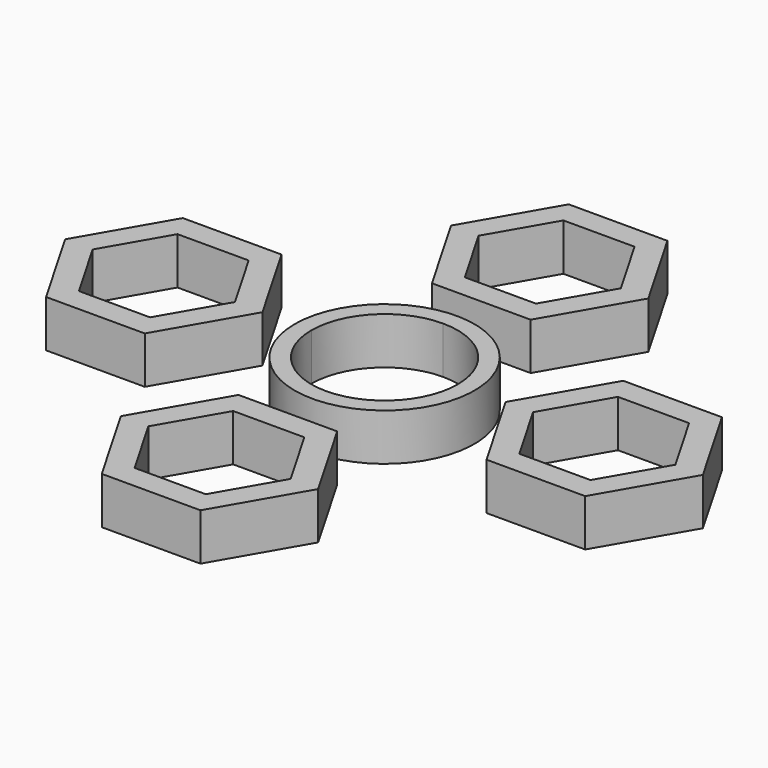
from build123d import *

# Parameters (mm, degrees)
F1_DEPTH = 7


# Not quite as in the source:
# - a feature names something its author has since deleted; it is built from what else it names


with BuildPart() as f1:
    # F0 (on Top) → F1 (new body)
    with BuildSketch(Plane.XY):
        Polygon((-25.5412213445, 12.7305734356), (-40.2412213445, 12.7305734356), (-47.5912213445, 0), (-40.2412213445, -12.7305734356), (-25.5412213445, -12.7305734356), (-18.1912213445, 0), align=None)
        Polygon((-43.4912213445, 0), (-38.1912213445, 9.1798692801), (-27.5912213445, 9.1798692801), (-22.2912213445, 0), (-27.5912213445, -9.1798692801), (-38.1912213445, -9.1798692801), align=None, mode=Mode.SUBTRACT)
    extrude(amount=F1_DEPTH)


with BuildPart() as f1b:
    # F0 (on Top) → F1, piece 2 (new body)
    with BuildSketch(Plane.XY):
        with BuildLine():
            ThreePointArc((-10.9, 0), (-7.7074639149, 7.7074639149), (0, 10.9))
            Line((0, 10.9), (0, 13.4))
            ThreePointArc((0, 13.4), (-9.4752308679, 9.4752308679), (-13.4, 0))
            Line((-13.4, 0), (-10.9, 0))
        make_face()
        with BuildLine():
            ThreePointArc((0, 10.9), (7.7074639149, 7.7074639149), (10.9, 0))
            Line((10.9, 0), (13.4, 0))
            ThreePointArc((13.4, 0), (9.4752308679, 9.4752308679), (0, 13.4))
            Line((0, 13.4), (0, 10.9))
        make_face()
        with BuildLine():
            Line((13.4, 0), (10.9, 0))
            ThreePointArc((10.9, 0), (7.7074639149, -7.7074639149), (0, -10.9))
            Line((0, -10.9), (0, -13.4))
            ThreePointArc((0, -13.4), (9.4752308679, -9.4752308679), (13.4, 0))
        make_face()
        with BuildLine():
            Line((0, -13.4), (0, -10.9))
            ThreePointArc((0, -10.9), (-7.7074639149, -7.7074639149), (-10.9, 0))
            Line((-10.9, 0), (-13.4, 0))
            ThreePointArc((-13.4, 0), (-9.4752308679, -9.4752308679), (0, -13.4))
        make_face()
    extrude(amount=F1_DEPTH)


with BuildPart() as f1c:
    # F0 (on Top) → F1, piece 3 (new body)
    with BuildSketch(Plane.XY):
        Polygon((7.35, -18.0137016425), (-7.35, -18.0137016425), (-14.7, -30.7442750782), (-7.35, -43.4748485138), (7.35, -43.4748485138), (14.7, -30.7442750782), align=None)
        Polygon((-10.6, -30.7442750782), (-5.3, -21.5644057981), (5.3, -21.5644057981), (10.6, -30.7442750782), (5.3, -39.9241443583), (-5.3, -39.9241443583), align=None, mode=Mode.SUBTRACT)
    extrude(amount=F1_DEPTH)


with BuildPart() as f1d:
    # F0 (on Top) → F1, piece 4 (new body)
    with BuildSketch(Plane.XY):
        Polygon((40.0694668353, 12.7305734356), (25.3694668353, 12.7305734356), (18.0194668353, 0), (25.3694668353, -12.7305734356), (40.0694668353, -12.7305734356), (47.4194668353, 0), align=None)
        Polygon((22.1194668353, 0), (27.4194668353, 9.1798692801), (38.0194668353, 9.1798692801), (43.3194668353, 0), (38.0194668353, -9.1798692801), (27.4194668353, -9.1798692801), align=None, mode=Mode.SUBTRACT)
    extrude(amount=F1_DEPTH)


with BuildPart() as f1e:
    # F0 (on Top) → F1, piece 5 (new body)
    with BuildSketch(Plane.XY):
        Polygon((7.35, 43.4748485138), (-7.35, 43.4748485138), (-14.7, 30.7442750782), (-7.35, 18.0137016425), (7.35, 18.0137016425), (14.7, 30.7442750782), align=None)
        Polygon((-10.6, 30.7442750782), (-5.3, 39.9241443583), (5.3, 39.9241443583), (10.6, 30.7442750782), (5.3, 21.5644057981), (-5.3, 21.5644057981), align=None, mode=Mode.SUBTRACT)
    extrude(amount=F1_DEPTH)


solid = Compound([f1.part, f1b.part, f1c.part, f1d.part, f1e.part])
